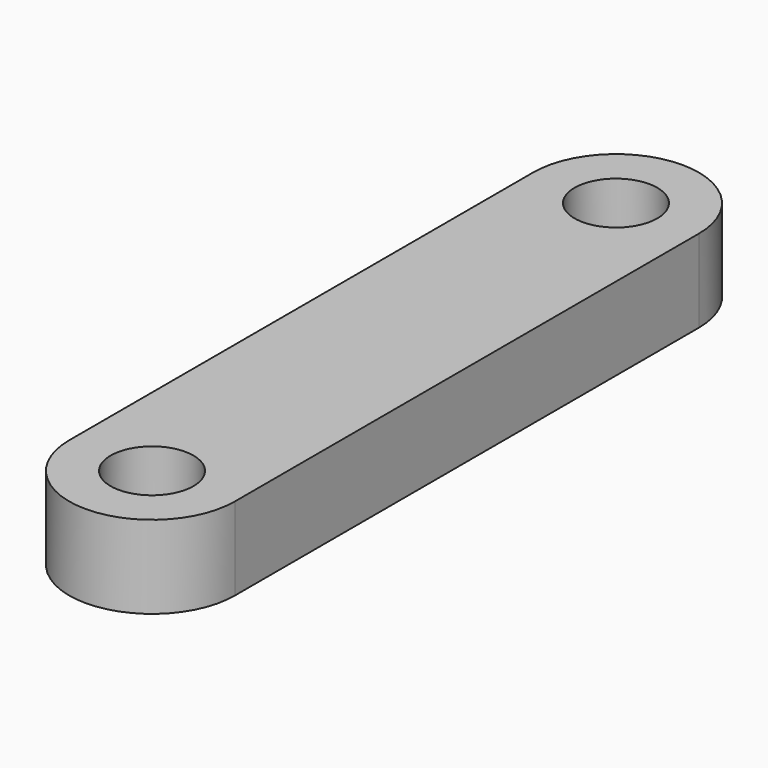
from build123d import *

# Parameters (mm, degrees)
F1_DEPTH = 25.4
F2_R     = 12.7
F3_DEPTH = 25.4


with BuildPart() as f1:
    # F0 (on Top) → F1 (new body)
    with BuildSketch(Plane.XY):
        with BuildLine():
            Line((-25.4, 88.9), (-25.4, 0))
            Line((-25.4, 0), (25.4, 0))
            Line((25.4, 0), (25.4, 88.9))
            ThreePointArc((25.4, 88.9), (0, 63.5), (-25.4, 88.9))
        make_face()
        with BuildLine():
            ThreePointArc((25.4, 88.9), (0, 114.3), (-25.4, 88.9))
            Line((-25.4, 88.9), (25.4, 88.9))
        make_face()
        with BuildLine():
            Line((25.4, 88.9), (-25.4, 88.9))
            ThreePointArc((-25.4, 88.9), (0, 63.5), (25.4, 88.9))
        make_face()
    extrude(amount=F1_DEPTH)

    # F2 (on face) → F3 (cut)
    with BuildSketch(Plane.XY.offset(25.4)):
        with Locations((0, 88.9)):
            Circle(F2_R)
    extrude(amount=-F3_DEPTH, mode=Mode.SUBTRACT)

    # F4: F1 across face


with BuildPart() as f1_1:
    add(f1.part)
    add(f1.part.mirror(Plane(origin=(0, 0, 12.7), x_dir=(1, 0, 0), z_dir=(0, -1, 0))))


solid = f1_1.part
